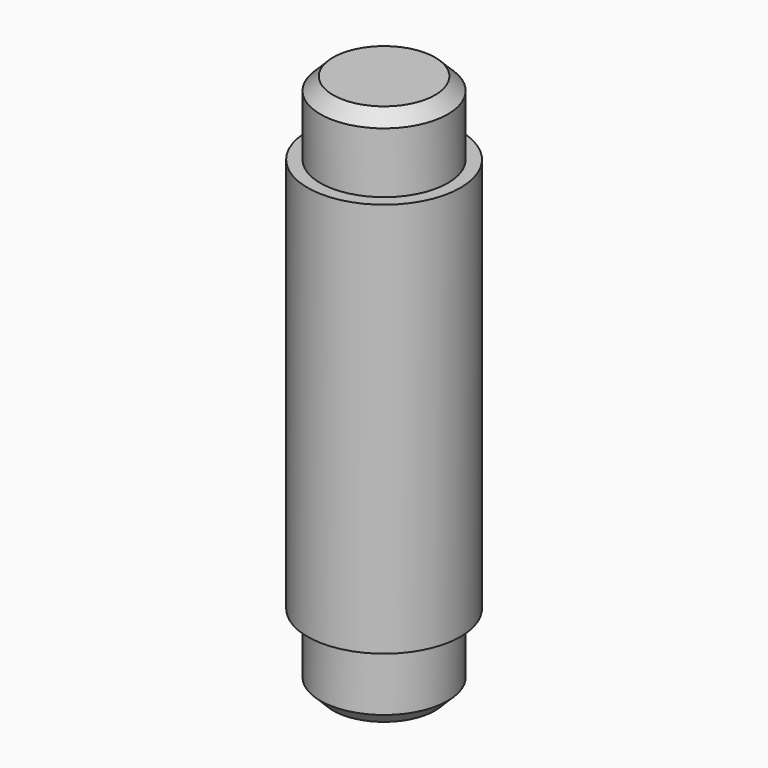
from build123d import *

# Parameters (mm, degrees)
F0_R     = 12
F1_DEPTH = 31
F2_R     = 10
F3_DEPTH = 11.5
F4_SIZE  = 2


# Not quite as in the source:
# - a pattern or mirror of a feature is missing from the dataset's text; its kind, count and spacing are read off the source's solid


with BuildPart() as f1:
    # F0 (on Top) → F1 (new body, symmetric)
    with BuildSketch(Plane.XY):
        Circle(F0_R)
    extrude(amount=F1_DEPTH, both=True)

    # F2 (on face) → F3 (join)
    with BuildSketch(Plane.XY.offset(31)):
        Circle(F2_R)
    f3 = extrude(amount=F3_DEPTH)

    # F3_copies: F3 across plane
    add(f3.mirror(Plane(origin=(0, 0, 0), x_dir=(-1, 0, 0), z_dir=(0, 0, -1))))

    # F4
    f4_edges = [f1.edges().sort_by_distance(p)[0] for p in [
        (-10, 0, 42.5),
        (-10, 0, -42.5),
    ]]
    chamfer(f4_edges, length=F4_SIZE)


solid = f1.part
